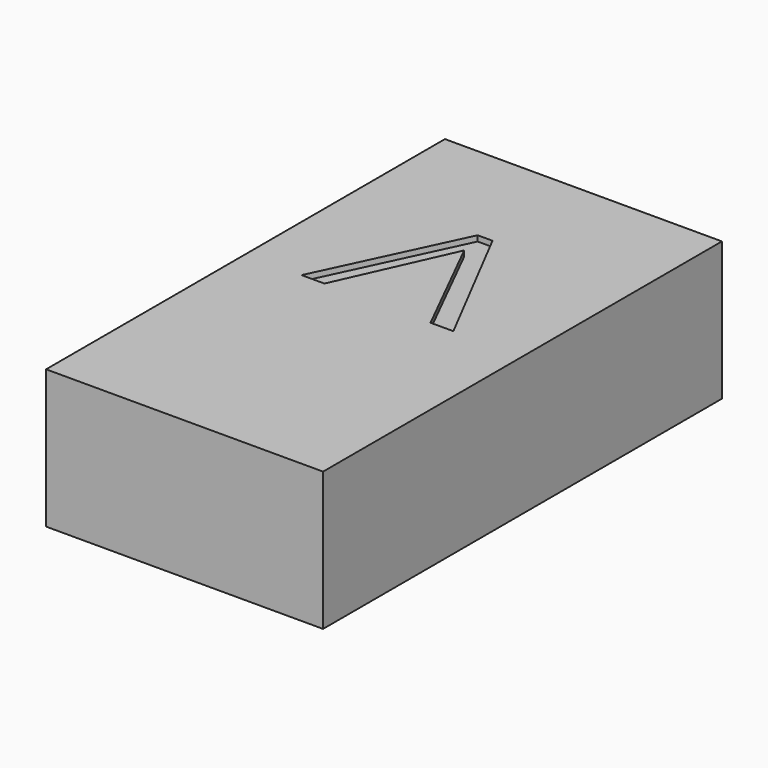
from build123d import *

# Parameters (mm, degrees)
F1_DEPTH     = 25
F2_TEXT_SIZE = 55.5555555556
F3_DEPTH     = 1


# Not quite as in the source:
# - Text() gives the source's letters only with a copy of the font that has no kerning and outlines rounded to 1/6400 em; it was checked with that copy


with BuildPart() as f1:
    # F0 (on Top) → F1 (new body)
    with BuildSketch(Plane.XY):
        Polygon((-25, 0), (0, 0), (25, 0), (25, 90), (0, 90), (-25, 90), align=None)
    extrude(amount=F1_DEPTH)

    # F2 (on face) → F3 (cut)
    with BuildSketch(Plane.XY.offset(25)):
        with Locations((-16.1631944444, 30)):
            Text('^', F2_TEXT_SIZE, font='Open Sans', text_align=(TextAlign.LEFT, TextAlign.BOTTOM))
    extrude(amount=-F3_DEPTH, mode=Mode.SUBTRACT)


solid = f1.part
